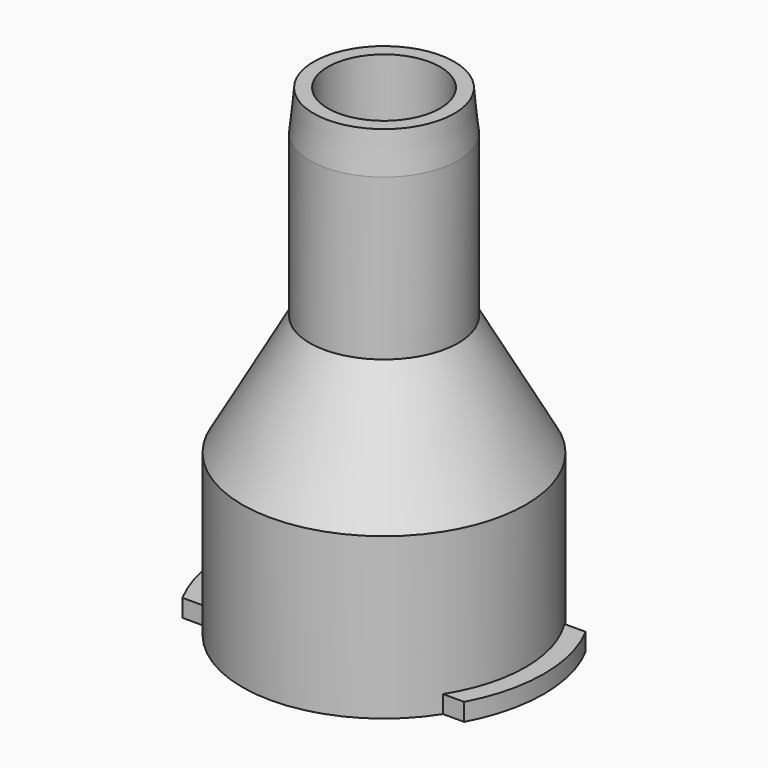
from build123d import *

# Parameters (mm, degrees)
F1_DEPTH = 2.2
F2_DEPTH = 20
F4_R     = 9.25
F4_R_2   = 7
F5_DEPTH = 25
F8_SIZE2 = 5
F8_SIZE  = 0.5


with BuildPart() as f1:
    # F0 (on Top) → F1 (new body)
    with BuildSketch(Plane.XY):
        with BuildLine():
            ThreePointArc((-14.9070453142, -9.45), (-17.65, 0), (-14.9070453142, 9.45))
            Line((-14.9070453142, 9.45), (-17.5414687241, 9.45))
            ThreePointArc((-17.5414687241, 9.45), (-19.925, 0), (-17.5414687241, -9.45))
            Line((-17.5414687241, -9.45), (-14.9070453142, -9.45))
        make_face()
        with BuildLine():
            ThreePointArc((14.9070453142, 9.45), (16.9503960101, 4.9200177949), (17.65, 0))
            ThreePointArc((17.65, 0), (16.9503960101, -4.9200177949), (14.9070453142, -9.45))
            Line((14.9070453142, -9.45), (17.5414687241, -9.45))
            ThreePointArc((17.5414687241, -9.45), (19.925, 0), (17.5414687241, 9.45))
            Line((17.5414687241, 9.45), (14.9070453142, 9.45))
        make_face()
        with BuildLine():
            Line((12.286069347, 9.45), (14.9070453142, 9.45))
            ThreePointArc((14.9070453142, 9.45), (0, 17.65), (-14.9070453142, 9.45))
            Line((-14.9070453142, 9.45), (-12.286069347, 9.45))
            ThreePointArc((-12.286069347, 9.45), (0, 15.5), (12.286069347, 9.45))
        make_face()
        with BuildLine():
            Line((-12.286069347, 9.45), (-14.9070453142, 9.45))
            ThreePointArc((-14.9070453142, 9.45), (-17.65, 0), (-14.9070453142, -9.45))
            Line((-14.9070453142, -9.45), (-12.286069347, -9.45))
            ThreePointArc((-12.286069347, -9.45), (-15.5, 0), (-12.286069347, 9.45))
        make_face()
        with BuildLine():
            ThreePointArc((-14.9070453142, -9.45), (0, -17.65), (14.9070453142, -9.45))
            Line((14.9070453142, -9.45), (12.286069347, -9.45))
            ThreePointArc((12.286069347, -9.45), (0, -15.5), (-12.286069347, -9.45))
            Line((-12.286069347, -9.45), (-14.9070453142, -9.45))
        make_face()
        with BuildLine():
            ThreePointArc((14.9070453142, -9.45), (16.9503960101, -4.9200177949), (17.65, 0))
            ThreePointArc((17.65, 0), (16.9503960101, 4.9200177949), (14.9070453142, 9.45))
            Line((14.9070453142, 9.45), (12.286069347, 9.45))
            ThreePointArc((12.286069347, 9.45), (14.6745370434, 4.9907877695), (15.5, 0))
            ThreePointArc((15.5, 0), (14.6745370434, -4.9907877695), (12.286069347, -9.45))
            Line((12.286069347, -9.45), (14.9070453142, -9.45))
        make_face()
    extrude(amount=F1_DEPTH)

    # F0 (on Top) → F2 (join)
    with BuildSketch(Plane.XY):
        with BuildLine():
            Line((12.286069347, 9.45), (14.9070453142, 9.45))
            ThreePointArc((14.9070453142, 9.45), (0, 17.65), (-14.9070453142, 9.45))
            Line((-14.9070453142, 9.45), (-12.286069347, 9.45))
            ThreePointArc((-12.286069347, 9.45), (0, 15.5), (12.286069347, 9.45))
        make_face()
        with BuildLine():
            Line((-12.286069347, 9.45), (-14.9070453142, 9.45))
            ThreePointArc((-14.9070453142, 9.45), (-17.65, 0), (-14.9070453142, -9.45))
            Line((-14.9070453142, -9.45), (-12.286069347, -9.45))
            ThreePointArc((-12.286069347, -9.45), (-15.5, 0), (-12.286069347, 9.45))
        make_face()
        with BuildLine():
            ThreePointArc((-14.9070453142, -9.45), (0, -17.65), (14.9070453142, -9.45))
            Line((14.9070453142, -9.45), (12.286069347, -9.45))
            ThreePointArc((12.286069347, -9.45), (0, -15.5), (-12.286069347, -9.45))
            Line((-12.286069347, -9.45), (-14.9070453142, -9.45))
        make_face()
        with BuildLine():
            ThreePointArc((14.9070453142, -9.45), (16.9503960101, -4.9200177949), (17.65, 0))
            ThreePointArc((17.65, 0), (16.9503960101, 4.9200177949), (14.9070453142, 9.45))
            Line((14.9070453142, 9.45), (12.286069347, 9.45))
            ThreePointArc((12.286069347, 9.45), (14.6745370434, 4.9907877695), (15.5, 0))
            ThreePointArc((15.5, 0), (14.6745370434, -4.9907877695), (12.286069347, -9.45))
            Line((12.286069347, -9.45), (14.9070453142, -9.45))
        make_face()
    extrude(amount=F2_DEPTH)



with BuildPart() as f5:
    # F4 (on offset) → F5 (new body)
    with BuildSketch(Plane.XY.offset(35)):
        Circle(F4_R)
        Circle(F4_R_2, mode=Mode.SUBTRACT)
    extrude(amount=F5_DEPTH)


with BuildPart() as f1_1:
    add(f1.part)

    add(f5.part)  # F7 merges F5
    # F6 (on Right) → F7 (revolve)
    with BuildSketch(Plane.YZ):
        Polygon((-9.25, 35), (-17.65, 20), (-15.5, 20), (-7, 35), align=None)
    revolve(axis=Axis((0, 0, 18.8534432091), (0, 0, -1)))

    # F8
    f8_edges = [f1_1.edges().sort_by_distance(p)[0] for p in [
        (-9.25, 0, 60),
    ]]
    f8_side = f1_1.faces().sort_by_distance((-8.98837, 0, 60))[0]
    chamfer(f8_edges, length=F8_SIZE, length2=F8_SIZE2, reference=f8_side)


solid = f1_1.part
